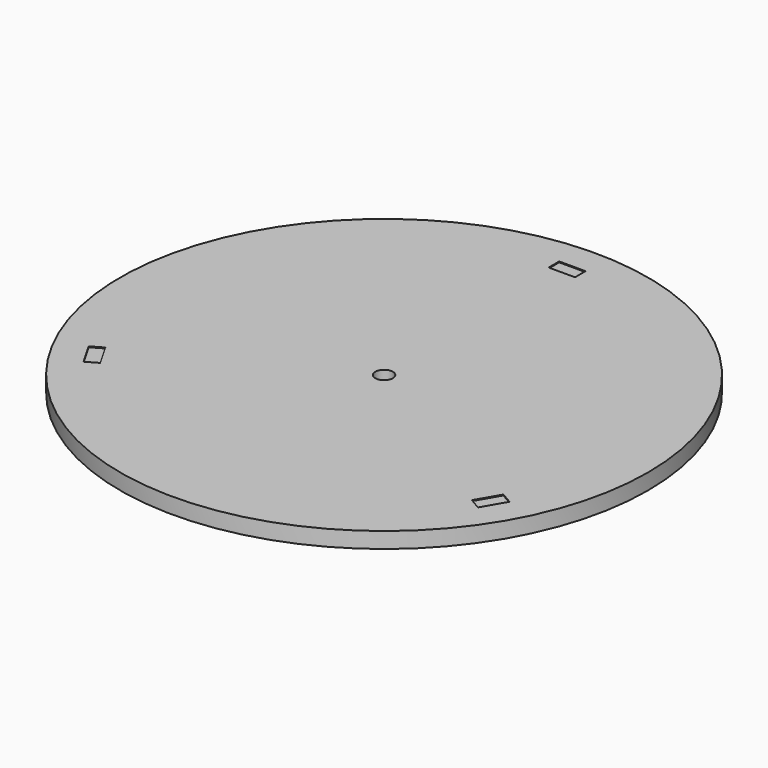
from build123d import *

# Parameters (mm, degrees)
F0_R            = 300
F0_R_2          = 10
F1_DEPTH        = 18
F2_R            = 2.5
F3_DEPTH        = 10
F3_COPIES_COUNT = 3
F4_W            = 60
F4_H            = 60
F5_DEPTH        = 2
F6_R            = 1
F7_DEPTH        = 5
F7_COPIES_COUNT = 4
F8_W            = 30
F8_H            = 15
F9_DEPTH        = 1
F9_COPIES_COUNT = 3


# Not quite as in the source:
# - a pattern or mirror of a feature is missing from the dataset's text; its kind, count and spacing are read off the source's solid


with BuildPart() as f1:
    # F0 (on Top) → F1 (new body)
    with BuildSketch(Plane.XY):
        Circle(F0_R)
        Circle(F0_R_2, mode=Mode.SUBTRACT)
    extrude(amount=F1_DEPTH)

    # F2 (on face) → F3 (cut)
    with BuildSketch(Plane(origin=(0, 0, 0), x_dir=(1, 0, 0), z_dir=(0, 0, -1))):
        with Locations((0, 250)):
            Circle(F2_R)
    f3 = extrude(amount=-F3_DEPTH, mode=Mode.SUBTRACT)

    # F3_copies: F3 ×3 about axis
    f3_copies_axis = Axis((0, 0, 0), (0, 0, 1))
    for i in range(1, F3_COPIES_COUNT):
        add(f3.rotate(f3_copies_axis, i * 360 / F3_COPIES_COUNT), mode=Mode.SUBTRACT)

    # F4 (on face) → F5 (cut)
    with BuildSketch(Plane(origin=(0, 0, 0), x_dir=(1, 0, 0), z_dir=(0, 0, -1))):
        Rectangle(F4_W, F4_H)
    extrude(amount=-F5_DEPTH, mode=Mode.SUBTRACT)

    # F6 (on face) → F7 (cut)
    with BuildSketch(Plane(origin=(0, 0, 2), x_dir=(1, 0, 0), z_dir=(0, 0, -1))):
        with Locations((21.2132034356, 21.2132034356)):
            Circle(F6_R)
    f7 = extrude(amount=-F7_DEPTH, mode=Mode.SUBTRACT)

    # F7_copies: F7 ×4 about axis
    f7_copies_axis = Axis((0, 0, 0), (0, 0, 1))
    for i in range(1, F7_COPIES_COUNT):
        add(f7.rotate(f7_copies_axis, i * 360 / F7_COPIES_COUNT), mode=Mode.SUBTRACT)

    # F8 (on face) → F9 (cut)
    with BuildSketch(Plane.XY.offset(18)):
        with Locations((0, 260)):
            Rectangle(F8_W, F8_H)
    f9 = extrude(amount=-F9_DEPTH, mode=Mode.SUBTRACT)

    # F9_copies: F9 ×3 about axis
    f9_copies_axis = Axis((0, 0, 0), (0, 0, 1))
    for i in range(1, F9_COPIES_COUNT):
        add(f9.rotate(f9_copies_axis, i * 360 / F9_COPIES_COUNT), mode=Mode.SUBTRACT)


solid = f1.part
